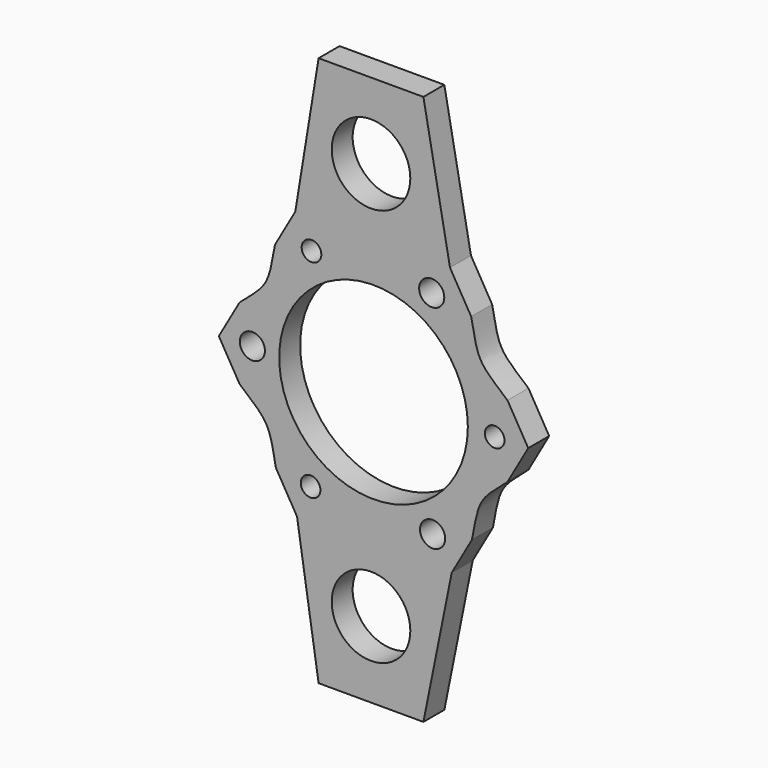
from build123d import *

# Parameters (mm, degrees)
F0_R     = 19.05
F0_R_2   = 4.7625
F0_R_3   = 6.096
F0_R_4   = 45.72
F1_DEPTH = 12.7


# Not quite as in the source:
# - ends of sketch curves that miss each other by under 0.0002 mm in the source are joined


with BuildPart() as f1:
    # F0 (on Front) → F1 (new body)
    with BuildSketch(Plane.XZ):
        with BuildLine():
            Line((37.0673326191, 65.1785315794), (24.1799304387, 133.8380140911))
            Line((24.1799304387, 133.8380140911), (-26.6200695613, 133.8380140911))
            Line((-26.6200695613, 133.8380140911), (-37.9125978196, 64.6905174884))
            Line((-37.9125978196, 64.6905174884), (-47.7326956793, 47.4230339812))
            add(Edge.make_bspline(
                [(-47.7326956793, 47.4230339812), (-51.0448461758, 29.0294404336), (-51.0448462531, 29.0294404776), (-64.9358999582, 17.1732288977)],
                knots=[0, 0, 0, 0, 34.7994388611, 34.7994388611, 34.7994388611, 34.7994388611], degree=3))
            Line((-64.9358999582, 17.1732288977), (-74.9799305502, -0.4880138996))
            Line((-74.9799305502, -0.4880138996), (-64.9359000035, -17.6262099378))
            add(Edge.make_bspline(
                [(-64.9359000035, -17.6262099378), (-50.6626559715, -29.6914131837), (-50.6626551721, -29.6914132451), (-47.3404022927, -47.649524558)],
                knots=[0, 0, 0, 0, 34.7994390827, 34.7994390827, 34.7994390827, 34.7994390827], degree=3))
            Line((-47.3404022927, -47.649524558), (-37.0673327313, -65.1785313884))
            Line((-37.0673327313, -65.1785313884), (-26.6200695613, -132.8619859089))
            Line((-26.6200695613, -132.8619859089), (24.1799304387, -132.8619859089))
            Line((24.1799304387, -132.8619859089), (37.9125978196, -64.6905174884))
            Line((37.9125978196, -64.6905174884), (47.7326956902, -47.4230338593))
            add(Edge.make_bspline(
                [(64.9358998918, -17.1732287319), (51.0448461867, -29.0294403117), (51.0448461867, -29.0294403117), (47.7326956902, -47.4230338593)],
                knots=[0, 0, 0, 0, 34.7994388611, 34.7994388611, 34.7994388611, 34.7994388611], degree=3))
            Line((64.9358998918, -17.1732287319), (74.9799304387, 0.4880140911))
            Line((74.9799304387, 0.4880140911), (64.9358998918, 17.6262101292))
            add(Edge.make_bspline(
                [(47.3404022927, 47.649524558), (50.662655861, 29.6914133741), (50.662655861, 29.6914133741), (64.9358998918, 17.6262101292)],
                knots=[0, 0, 0, 0, 34.7994388611, 34.7994388611, 34.7994388611, 34.7994388611], degree=3))
            Line((47.3404022927, 47.649524558), (37.0673326191, 65.1785315794))
        make_face()
        with Locations((-1.2200695613, -96.0319859089)):
            Circle(F0_R, mode=Mode.SUBTRACT)
        with Locations((-30.4998691349, -50.180102728)):
            Circle(F0_R_2, mode=Mode.SUBTRACT)
        with Locations((28.6262483892, -51.2720453093)):
            Circle(F0_R_3, mode=Mode.SUBTRACT)
        Circle(F0_R_4, mode=Mode.SUBTRACT)
        with Locations((58.7220974339, 0)):
            Circle(F0_R_2, mode=Mode.SUBTRACT)
        with Locations((-58.7227720341, 0.4880365509)):
            Circle(F0_R_3, mode=Mode.SUBTRACT)
        with Locations((-30.0641650228, 50.4423503469)):
            Circle(F0_R_2, mode=Mode.SUBTRACT)
        with Locations((-1.2200695613, 97.0080140911)):
            Circle(F0_R, mode=Mode.SUBTRACT)
        with Locations((28.1997188878, 51.5078691239)):
            Circle(F0_R_3, mode=Mode.SUBTRACT)
    extrude(amount=F1_DEPTH)


solid = f1.part
